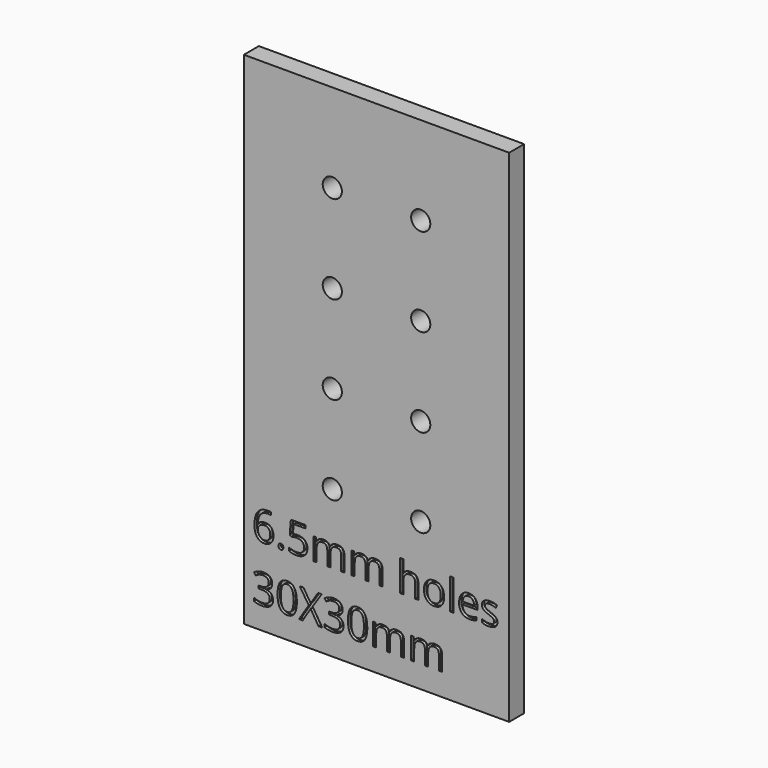
from build123d import *

# Parameters (mm, degrees)
F0_W         = 90
F0_H         = 170
F0_R         = 3.25
F1_DEPTH     = 6.35
F0_R_2       = 1.5
F3_TEXT_SIZE = 13.8888888889
F4_DEPTH     = 1


# Not quite as in the source:
# - Text() gives the source's letters only with a copy of the font that has no kerning and outlines rounded to 1/6400 em; it was checked with that copy


with BuildPart() as f1:
    # F0 (on Front) → F1 (new body)
    with BuildSketch(Plane.XZ):
        Rectangle(F0_W, F0_H)
        with Locations((-15, -35)):
            Circle(F0_R, mode=Mode.SUBTRACT)
        with Locations((-15, -5)):
            Circle(F0_R, mode=Mode.SUBTRACT)
        with Locations((15, -35)):
            Circle(F0_R, mode=Mode.SUBTRACT)
        with Locations((15, -5)):
            Circle(F0_R, mode=Mode.SUBTRACT)
        with Locations((-15, 25)):
            Circle(F0_R, mode=Mode.SUBTRACT)
        with Locations((15, 25)):
            Circle(F0_R, mode=Mode.SUBTRACT)
        with Locations((-15, 55)):
            Circle(F0_R, mode=Mode.SUBTRACT)
        with Locations((15, 55)):
            Circle(F0_R, mode=Mode.SUBTRACT)
    extrude(amount=F1_DEPTH)

    # F3 (on face) → F4 (cut)
    with BuildSketch(Plane.XZ.offset(6.35)):
        with Locations((-42.2153026565, -58.5770174503)):
            Text('6.5mm holes', F3_TEXT_SIZE, font='Open Sans', text_align=(TextAlign.LEFT, TextAlign.BOTTOM))
        with Locations((-42.2153026565, -77.4659063392)):
            Text('30X30mm', F3_TEXT_SIZE, font='Open Sans', text_align=(TextAlign.LEFT, TextAlign.BOTTOM))
    extrude(amount=-F4_DEPTH, mode=Mode.SUBTRACT)


with BuildPart() as f1b:
    # F0 (on Front) → F1, piece 2 (new body)
    with BuildSketch(Plane.XZ):
        with Locations((-415, 250)):
            Circle(F0_R_2)
    extrude(amount=F1_DEPTH)


solid = f1.part
